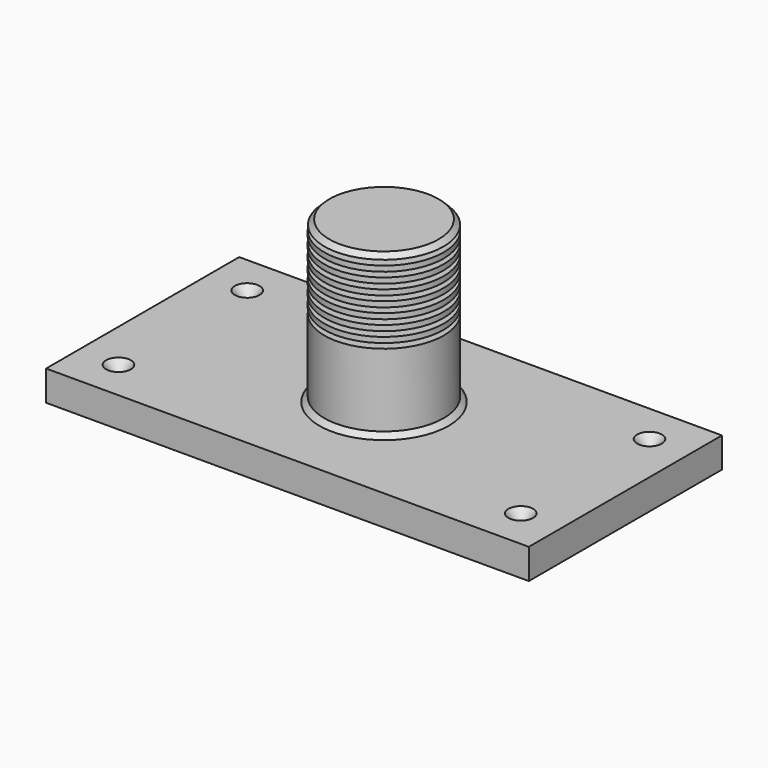
from build123d import *

# Parameters (mm, degrees)
F0_W           = 152.4
F0_H           = 76.2
F1_DEPTH       = 9.525
F3_D           = 2.7051
F3_CSINK_D     = 7.7978
F3_CSINK_ANGLE = 82
F4_R           = 18.8204674016
F5_DEPTH       = 50.8
F6_W           = 14.3435228881
F6_H           = 1.5875


# Not quite as in the source:
# - a fillet or chamfer that OpenCascade refuses, or shapes differently, is made with other operations: its cross-section is extruded or revolved along the edge and cut away or added


with BuildPart() as f1:
    # F0 (on Top) → F1 (new body)
    with BuildSketch(Plane.XY):
        Rectangle(F0_W, F0_H)
    extrude(amount=F1_DEPTH)

    # F3 (through all)
    with Locations(Plane.XY.offset(9.525)):
        with Locations((-63.5, 25.4), (63.5, 25.4), (-63.5, -25.4), (63.5, -25.4)):
            CounterSinkHole(F3_D / 2, F3_CSINK_D / 2, counter_sink_angle=F3_CSINK_ANGLE)

    # F4 (on face) → F5 (join)
    with BuildSketch(Plane.XY.offset(9.525)):
        Circle(F4_R)
    extrude(amount=F5_DEPTH)

    # F6 (on Front) → F7 (revolve, cut)
    with BuildSketch(Plane.XZ):
        with Locations((19.8717614441, 34.8877100782)):
            Rectangle(F6_W, F6_H)
        with Locations((19.8717614441, 38.1897100782)):
            Rectangle(F6_W, F6_H)
        with Locations((19.8717614441, 41.4917100782)):
            Rectangle(F6_W, F6_H)
        with Locations((19.8717614441, 44.7937100782)):
            Rectangle(F6_W, F6_H)
        with Locations((19.8717614441, 48.0957100782)):
            Rectangle(F6_W, F6_H)
        with Locations((19.8717614441, 51.3977100782)):
            Rectangle(F6_W, F6_H)
        with Locations((19.8717614441, 54.6997100782)):
            Rectangle(F6_W, F6_H)
        with Locations((19.8717614441, 58.0017100782)):
            Rectangle(F6_W, F6_H)
    revolve(axis=Axis((0, 0, 9.525), (0, 0, -1)), mode=Mode.SUBTRACT)

    # F8: chamfer of 1.5875 on 2 edges, made by hand

    # F8_s1 → F8_t2 (revolve)
    with BuildSketch(Plane.XZ):
        Polygon((20.4079674016, 9.525), (18.8204674016, 11.1125), (18.8204674016, 9.525), align=None)
    revolve(axis=Axis((0, 0, 9.525), (0, 0, 1)))

    # F8_s3 → F8_t4 (revolve, cut)
    with BuildSketch(Plane.XZ):
        Polygon((18.8204674016, 58.7375), (17.2329674016, 60.325), (18.8204674016, 60.325), align=None)
    revolve(axis=Axis((0, 0, 60.325), (0, 0, 1)), mode=Mode.SUBTRACT)


solid = f1.part
